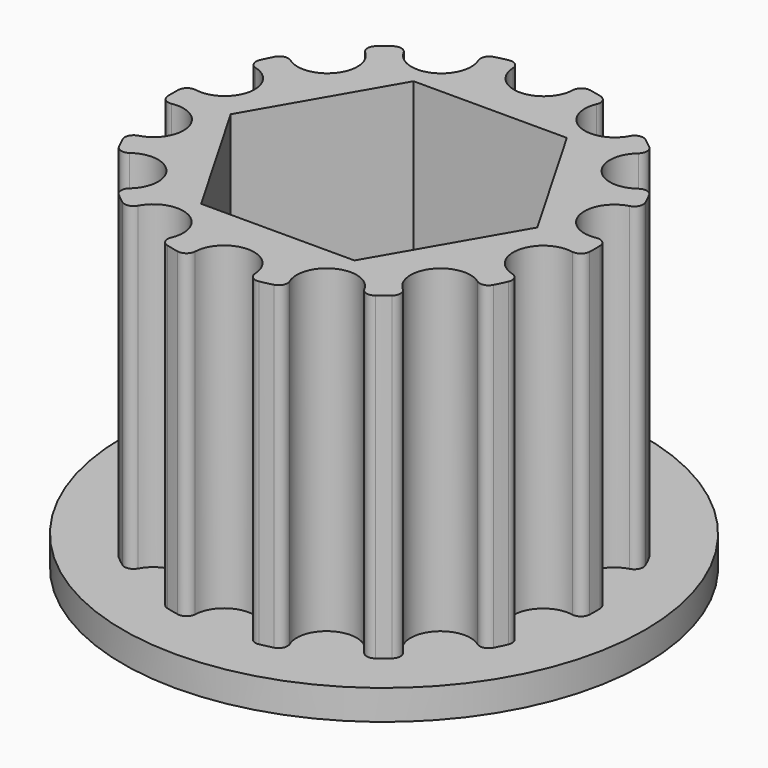
from build123d import *

# Parameters (mm, degrees)
F2_R            = 10.5683460292
F3_DEPTH        = 16
F5_DEPTH        = 16
F5_COPIES_COUNT = 14
F8_R            = 13.0683460292
F8_R_2          = 10.5683460292
F9_DEPTH        = 1.5
F10_DEPTH       = 17.501


# Not quite as in the source:
# - a feature of the source that left no trace in its solid (it failed there, or was rolled back) is left out
# - a pattern or mirror of a feature is missing from the dataset's text; its kind, count and spacing are read off the source's solid


with BuildPart() as f3:
    # F2 (on Top) → F3 (new body)
    with BuildSketch(Plane.XY):
        Circle(F2_R)
    extrude(amount=F3_DEPTH)

    # F4 (on face) → F5 (cut, through all)
    with BuildSketch(Plane.XY.offset(16)):
        with BuildLine():
            ThreePointArc((-2.035036184, 10.3705624496), (-1.6695907294, 10.2822178496), (-1.4987572129, 9.9472983692))
            ThreePointArc((-1.4987572129, 9.9472983692), (0, 8.5083460292), (1.4987572129, 9.9472983692))
            ThreePointArc((1.4987572129, 9.9472983692), (1.6695907294, 10.2822178496), (2.035036184, 10.3705624496))
            ThreePointArc((2.035036184, 10.3705624496), (0, 10.5683460292), (-2.035036184, 10.3705624496))
        make_face()
    f5 = extrude(amount=-F5_DEPTH, mode=Mode.SUBTRACT)

    # F5_copies: F5 ×14 about axis
    f5_copies_axis = Axis((0, 0, 0), (0, 0, 1))
    for i in range(1, F5_COPIES_COUNT):
        add(f5.rotate(f5_copies_axis, i * 360 / F5_COPIES_COUNT), mode=Mode.SUBTRACT)

    # F8 (on face) + F2 (on Top) → F9 (join)
    with BuildSketch(Plane.XY):
        Circle(F8_R)
        Circle(F8_R_2, mode=Mode.SUBTRACT)
    with BuildSketch(Plane.XY):
        Circle(F2_R)
    extrude(amount=-F9_DEPTH)

    # F7 (on face) → F10 (cut, through all)
    with BuildSketch(Plane.XY.offset(16)):
        Polygon((3.8393792901, 6.65), (-3.8393792901, 6.65), (-7.6787585802, 0), (-3.8393792901, -6.65), (3.8393792901, -6.65), (7.6787585802, 0), align=None)
    extrude(amount=-F10_DEPTH, mode=Mode.SUBTRACT)


solid = f3.part
